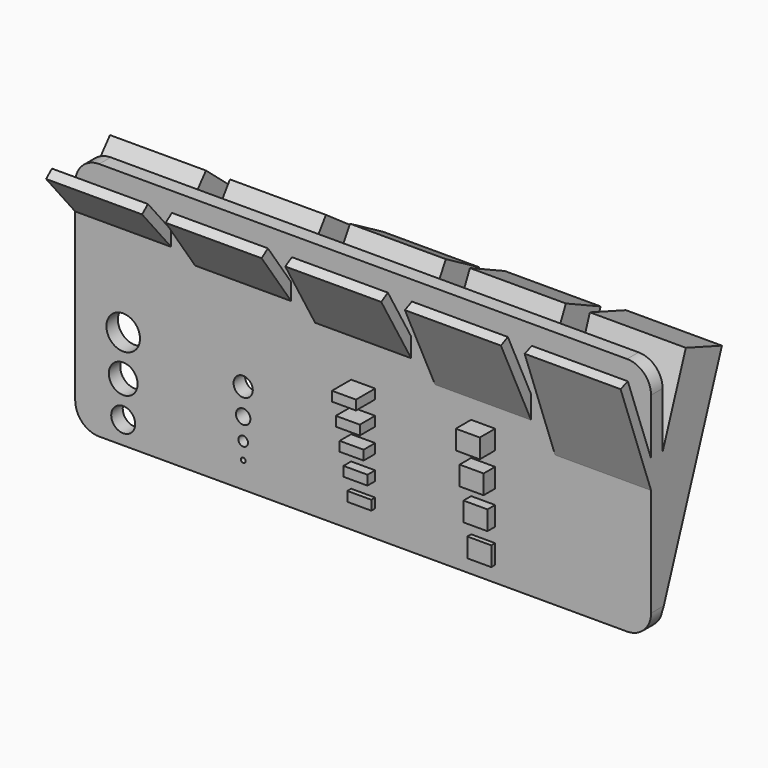
from build123d import *

# Parameters (mm, degrees)
F0_W          = 58.5
F0_H          = 1.5
F0_H_2        = 3
F1_DEPTH      = 50
F9_DEPTH      = 10
F10_T1_DEPTH  = 28
F10_T3_DEPTH  = 14
F10_T5_DEPTH  = 14
F10_T10_DEPTH = 28
F10_T16_DEPTH = 28
F11_R         = 0.5
F11_R_2       = 1
F11_R_3       = 1.5
F11_R_4       = 2
F11_R_5       = 2.5
F11_R_6       = 3
F11_R_7       = 3.5
F12_DEPTH     = 3
F13_W         = 5
F13_H         = 2
F14_W         = 5
F14_H         = 4
F15_DEPTH     = 1
F16_DEPTH     = 2
F17_DEPTH     = 3
F18_DEPTH     = 4
F19_DEPTH     = 5


# Not quite as in the source:
# - a fillet or chamfer that OpenCascade refuses, or shapes differently, is made with other operations: its cross-section is extruded or revolved along the edge and cut away or added


with BuildPart() as f1:
    # F0 (on Top) → F1 (new body)
    with BuildSketch(Plane.XY):
        with Locations((-30.75, -0.75)):
            Rectangle(F0_W, F0_H)
        with Locations((-30.75, 0.75)):
            Rectangle(F0_W, F0_H)
        Polygon((1.5, 1.5), (-1.5, 1.5), (-1.5, 0), (-1.5, -1.5), (1.5, -1.5), align=None)
        with Locations((30.75, 0)):
            Rectangle(F0_W, F0_H_2)
    extrude(amount=F1_DEPTH)

    # F4 (on offset) + F5 (on offset) + F6 (on Right) + F7 (on face) + F8 (on face) → F9 (join, symmetric)
    with BuildSketch(Plane.YZ.offset(50)):
        Polygon((0, 23.3904352013), (0, 0), (16.9536601964, 46.5797985667), (7.5567339886, 50), (0, 29.2380440016), align=None)
        Polygon((-9.4361192301, 49.3159597133), (0, 23.3904352013), (0, 29.2380440016), (-7.5567339886, 50), align=None)
    with BuildSketch(Plane.YZ.offset(25)):
        Polygon((0, 29.0621284988), (0, 10.1325158336), (16.6198118589, 45.7738173826), (7.5567339886, 50), (0, 33.7945316651), align=None)
        Polygon((-9.3693495626, 49.1547634765), (0, 29.0621284988), (0, 33.7945316651), (-7.5567339886, 50), align=None)
    with BuildSketch(Plane.YZ):
        Polygon((0, 32.9113527925), (0, 16.9113527925), (16.2169880264, 45), (7.5567339886, 50), (0, 36.9113527925), align=None)
        Polygon((-9.2887847961, 49), (0, 32.9113527925), (0, 36.9113527925), (-7.5567339886, 50), align=None)
    with BuildSketch(Plane(origin=(-25, 0, 0), x_dir=(0, -1, 0), z_dir=(-1, 0, 0))):
        Polygon((-15.7482544314, 44.2642356365), (0, 21.7733974606), (0, 35.7209718255), (0, 39.2078654168), (-7.5567339886, 50), align=None)
        Polygon((0, 39.2078654168), (0, 35.7209718255), (9.1950380771, 48.8528471273), (7.5567339886, 50), align=None)
    with BuildSketch(Plane(origin=(-50, 0, 0), x_dir=(0, -1, 0), z_dir=(-1, 0, 0))):
        Polygon((-15.2171784197, 43.5721239031), (0, 25.4369968523), (0, 37.8827874671), (0, 40.9942351209), (-7.5567339886, 50), align=None)
        Polygon((0, 40.9942351209), (0, 37.8827874671), (9.0888228748, 48.7144247806), (7.5567339886, 50), align=None)
    extrude(amount=F9_DEPTH, both=True, dir=(1, 0, 0))

    # F10: fillet of radius 5 on 5 edges, made by hand

    # F10_s2 → F10_t1 (cut)
    with BuildSketch(Plane.XZ.offset(-14)):
        with BuildLine():
            ThreePointArc((-55, 0), (-58.5355339059, 1.4644660941), (-60, 5))
            Line((-60, 5), (-60, 0))
            Line((-60, 0), (-55, 0))
        make_face()
    extrude(amount=F10_T1_DEPTH, mode=Mode.SUBTRACT)

    # F10_s4 → F10_t3 (cut)
    with BuildSketch(Plane.XZ):
        with BuildLine():
            ThreePointArc((55, 0), (58.5355339059, 1.4644660941), (60, 5))
            Line((60, 5), (60, 0))
            Line((60, 0), (55, 0))
        make_face()
    extrude(amount=F10_T3_DEPTH, mode=Mode.SUBTRACT)

    # F10_s6 → F10_t5 (cut)
    with BuildSketch(Plane.XZ.offset(-14)):
        with BuildLine():
            ThreePointArc((55, 0), (58.5355339059, 1.4644660941), (60, 5))
            Line((60, 5), (60, 0))
            Line((60, 0), (55, 0))
        make_face()
    extrude(amount=F10_T5_DEPTH, mode=Mode.SUBTRACT)


with BuildPart() as f10_tool8:
    # F10_s9 → F10_t10 (new body)
    with BuildSketch(Plane.XZ.offset(14)):
        with BuildLine():
            ThreePointArc((60, 45), (58.5355339059, 48.5355339059), (55, 50))
            Line((55, 50), (60, 50))
            Line((60, 50), (60, 45))
        make_face()
    extrude(amount=-F10_T10_DEPTH)

    split(bisect_by=Plane(origin=(0, 9.3969262079, 3.4202014333), x_dir=(1, 0, 0), z_dir=(0, 0.9396926208, 0.3420201433)), keep=Keep.TOP)

    split(bisect_by=Plane(origin=(0, -9.3969262079, 3.4202014333), x_dir=(1, 0, 0), z_dir=(0, -0.9396926208, 0.3420201433)), keep=Keep.TOP)


with BuildPart() as f1_1:
    add(f1.part)

    # F10_t7: cut F10_tool8
    add(f10_tool8.part, mode=Mode.SUBTRACT)


with BuildPart() as f10_tool14:
    # F10_s15 → F10_t16 (new body)
    with BuildSketch(Plane.XZ.offset(-14)):
        with BuildLine():
            ThreePointArc((-55, 50), (-58.5355339059, 48.5355339059), (-60, 45))
            Line((-60, 45), (-60, 50))
            Line((-60, 50), (-55, 50))
        make_face()
    extrude(amount=F10_T16_DEPTH)

    split(bisect_by=Plane(origin=(0, 20.1857202879, 16.9378304486), x_dir=(1, 0, 0), z_dir=(0, 0.7660444431, 0.6427876097)), keep=Keep.TOP)

    split(bisect_by=Plane(origin=(0, -20.1857202879, 16.9378304486), x_dir=(1, 0, 0), z_dir=(0, -0.7660444431, 0.6427876097)), keep=Keep.TOP)


with BuildPart() as f1_2:
    add(f1_1.part)

    # F10_t13: cut F10_tool14
    add(f10_tool14.part, mode=Mode.SUBTRACT)

    # F11 (on face) → F12 (cut, through all)
    with BuildSketch(Plane(origin=(0, 1.5, 0), x_dir=(-1, 0, 0), z_dir=(0, 1, 0))):
        with Locations((25, 5.4156194707)):
            Circle(F11_R)
        with Locations((25, 8.9156194707)):
            Circle(F11_R_2)
        with Locations((25, 13.4156194707)):
            Circle(F11_R_3)
        with Locations((25, 18.9156194707)):
            Circle(F11_R_4)
        with Locations((50, 4.7246272412)):
            Circle(F11_R_5)
        with Locations((50, 12.2246272412)):
            Circle(F11_R_6)
        with Locations((50, 20.7246272412)):
            Circle(F11_R_7)
    extrude(amount=-F12_DEPTH, mode=Mode.SUBTRACT)

    # F13 (on face) + F14 (on face) → F15 (join)
    with BuildSketch(Plane.XZ.offset(1.5)):
        with Locations((0, 6.5094290039)):
            Rectangle(F13_W, F13_H)
    with BuildSketch(Plane.XZ.offset(1.5)):
        with Locations((25, 5.2788888796)):
            Rectangle(F14_W, F14_H)
    extrude(amount=F15_DEPTH)

    # F13 (on face) + F14 (on face) → F16 (join)
    with BuildSketch(Plane.XZ.offset(1.5)):
        with Locations((0, 11.5094290039)):
            Rectangle(F13_W, F13_H)
    with BuildSketch(Plane.XZ.offset(1.5)):
        with Locations((25, 12.2788888796)):
            Rectangle(F14_W, F14_H)
    extrude(amount=F16_DEPTH)

    # F13 (on face) + F14 (on face) → F17 (join)
    with BuildSketch(Plane.XZ.offset(1.5)):
        with Locations((0, 16.5094290039)):
            Rectangle(F13_W, F13_H)
    with BuildSketch(Plane.XZ.offset(1.5)):
        with Locations((25, 19.2788888796)):
            Rectangle(F14_W, F14_H)
    extrude(amount=F17_DEPTH)

    # F13 (on face) + F14 (on face) → F18 (join)
    with BuildSketch(Plane.XZ.offset(1.5)):
        with Locations((0, 21.5094290039)):
            Rectangle(F13_W, F13_H)
    with BuildSketch(Plane.XZ.offset(1.5)):
        with Locations((25, 26.2788888796)):
            Rectangle(F14_W, F14_H)
    extrude(amount=F18_DEPTH)

    # F13 (on face) → F19 (join)
    with BuildSketch(Plane.XZ.offset(1.5)):
        with Locations((0, 26.5094290039)):
            Rectangle(F13_W, F13_H)
    extrude(amount=F19_DEPTH)


solid = f1_2.part
